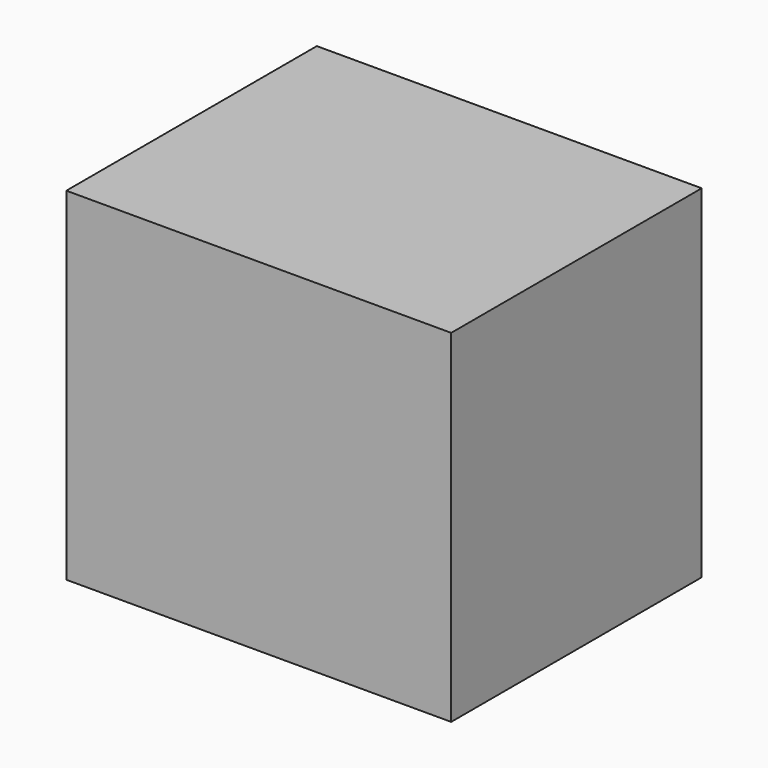
from build123d import *

# Parameters (mm, degrees)
F0_W     = 31.2210861593
F0_H     = 27.783902362
F1_DEPTH = 25.4


# Not quite as in the source:
# - the program builds the solid bodies; features that only make, move or delete a surface that nothing else refers to are left out


with BuildPart() as f1:
    # F0 (on Front) → F1 (new body)
    with BuildSketch(Plane.XZ):
        with Locations((-15.6105430797, 13.891951181)):
            Rectangle(F0_W, F0_H)
    extrude(amount=F1_DEPTH)


solid = f1.part
